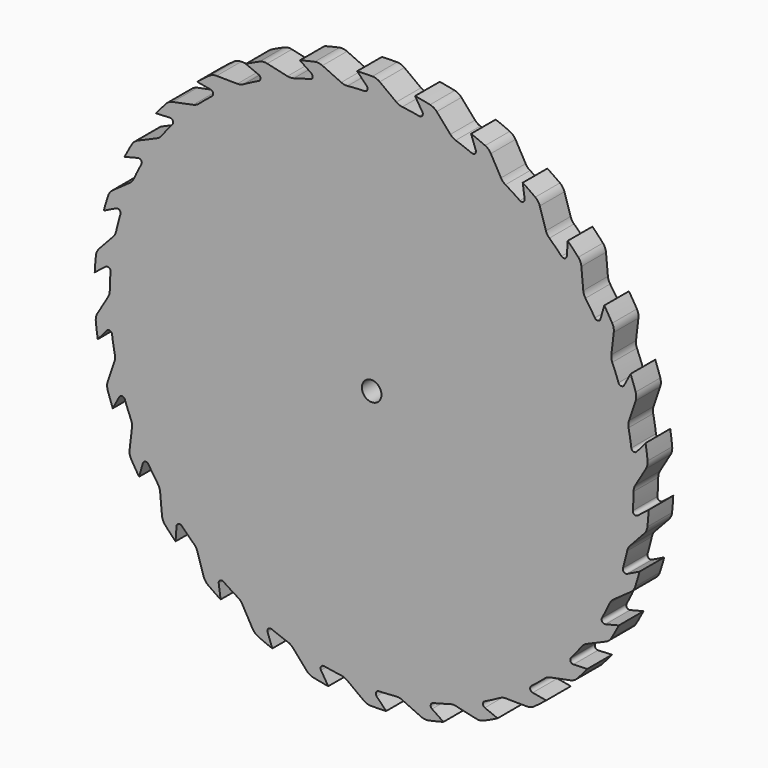
from build123d import *

# Parameters (mm, degrees)
F0_R            = 45
F1_DEPTH        = 5
F4_DEPTH        = 25
F4_COPIES_COUNT = 30
F5_R            = 2
F6_R            = 0.5
F7_R            = 1.5875
F8_DEPTH        = 25


# Not quite as in the source:
# - a pattern or mirror of a feature is missing from the dataset's text; its kind, count and spacing are read off the source's solid


with BuildPart() as f1:
    # F0 (on Front) → F1 (new body)
    with BuildSketch(Plane.XZ):
        Circle(F0_R)
    extrude(amount=F1_DEPTH)

    # F2 (on face) → F4 (cut)
    with BuildSketch(Plane.XZ.offset(5)):
        with BuildLine():
            Line((-8.5864047919, 44.1732232551), (-4.4424596889, 42.2671805532))
            ThreePointArc((-4.4424596889, 42.2671805532), (-2.2242781403, 42.4417552271), (0, 42.5))
            Line((0, 42.5), (-2.3551180309, 44.938329064))
            ThreePointArc((-2.3551180309, 44.938329064), (-5.4841204532, 44.6645768239), (-8.5864047919, 44.1732232551))
        make_face()
    f4 = extrude(amount=-F4_DEPTH, mode=Mode.SUBTRACT)

    # F4_copies: F4 ×30 about axis
    f4_copies_axis = Axis((0, 0, 0), (0, 1, 0))
    for i in range(1, F4_COPIES_COUNT):
        add(f4.rotate(f4_copies_axis, i * 360 / F4_COPIES_COUNT), mode=Mode.SUBTRACT)

    # F5
    f5_edges = [f1.edges().sort_by_distance(p)[0] for p in [
        (-8.586405, -2.5, 44.173223),
        (-4.44246, -2.5, 42.267181),
        (0.785358, -2.5, 44.993146),
        (4.44246, -2.5, 42.267181),
        (10.122797, -2.5, 43.846653),
        (13.133222, -2.5, 40.419902),
        (19.017822, -2.5, 40.78385),
        (21.25, -2.5, 36.80608),
        (27.081676, -2.5, 35.938598),
        (28.438051, -2.5, 31.583655),
        (33.961931, -2.5, 29.522656),
        (34.383222, -2.5, 24.980873),
        (39.357887, -2.5, 21.816433),
        (38.825682, -2.5, 17.286307),
        (43.033714, -2.5, 13.156727),
        (41.571273, -2.5, 8.836247),
        (44.828761, -2.5, 3.922008),
        (42.5, -2.5, 0),
        (44.664577, -2.5, -5.48412),
        (41.571273, -2.5, -8.836247),
        (42.548336, -2.5, -14.650567),
        (38.825682, -2.5, -17.286307),
        (38.572529, -2.5, -23.176713),
        (34.383222, -2.5, -24.980873),
        (32.910917, -2.5, -30.689926),
        (28.438051, -2.5, -31.583655),
        (25.81094, -2.5, -36.861842),
        (21.25, -2.5, -36.80608),
        (17.582901, -2.5, -41.422718),
        (13.133222, -2.5, -40.419902),
        (8.586405, -2.5, -44.173223),
        (4.44246, -2.5, -42.267181),
        (-0.785358, -2.5, -44.993146),
        (-4.44246, -2.5, -42.267181),
        (-10.122797, -2.5, -43.846653),
        (-13.133222, -2.5, -40.419902),
        (-19.017822, -2.5, -40.78385),
        (-21.25, -2.5, -36.80608),
        (-27.081676, -2.5, -35.938598),
        (-28.438051, -2.5, -31.583655),
        (-33.961931, -2.5, -29.522656),
        (-34.383222, -2.5, -24.980873),
        (-39.357887, -2.5, -21.816433),
        (-38.825682, -2.5, -17.286307),
        (-43.033714, -2.5, -13.156727),
        (-41.571273, -2.5, -8.836247),
        (-44.828761, -2.5, -3.922008),
        (-42.5, -2.5, 0),
        (-44.664577, -2.5, 5.48412),
        (-41.571273, -2.5, 8.836247),
        (-42.548336, -2.5, 14.650567),
        (-38.825682, -2.5, 17.286307),
        (-38.572529, -2.5, 23.176713),
        (-34.383222, -2.5, 24.980873),
        (-32.910917, -2.5, 30.689926),
        (-28.438051, -2.5, 31.583655),
        (-25.81094, -2.5, 36.861842),
        (-21.25, -2.5, 36.80608),
        (-17.582901, -2.5, 41.422718),
        (-13.133222, -2.5, 40.419902),
    ]]
    fillet(f5_edges, radius=F5_R)

    # F6
    f6_edges = [f1.edges().sort_by_distance(p)[0] for p in [
        (0, -2.5, 42.5),
        (-8.836247, -2.5, 41.571273),
        (8.836247, -2.5, 41.571273),
        (-17.286307, -2.5, 38.825682),
        (17.286307, -2.5, 38.825682),
        (-24.980873, -2.5, 34.383222),
        (24.980873, -2.5, 34.383222),
        (-31.583655, -2.5, 28.438051),
        (31.583655, -2.5, 28.438051),
        (-36.80608, -2.5, 21.25),
        (36.80608, -2.5, 21.25),
        (-40.419902, -2.5, 13.133222),
        (40.419902, -2.5, 13.133222),
        (-42.267181, -2.5, 4.44246),
        (42.267181, -2.5, 4.44246),
        (-42.267181, -2.5, -4.44246),
        (42.267181, -2.5, -4.44246),
        (-40.419902, -2.5, -13.133222),
        (40.419902, -2.5, -13.133222),
        (-36.80608, -2.5, -21.25),
        (36.80608, -2.5, -21.25),
        (-31.583655, -2.5, -28.438051),
        (31.583655, -2.5, -28.438051),
        (-24.980873, -2.5, -34.383222),
        (24.980873, -2.5, -34.383222),
        (-17.286307, -2.5, -38.825682),
        (17.286307, -2.5, -38.825682),
        (-8.836247, -2.5, -41.571273),
        (8.836247, -2.5, -41.571273),
        (0, -2.5, -42.5),
    ]]
    fillet(f6_edges, radius=F6_R)

    # F7 (on face) → F8 (cut)
    with BuildSketch(Plane.XZ.offset(5)):
        Circle(F7_R)
    extrude(amount=-F8_DEPTH, mode=Mode.SUBTRACT)


solid = f1.part
